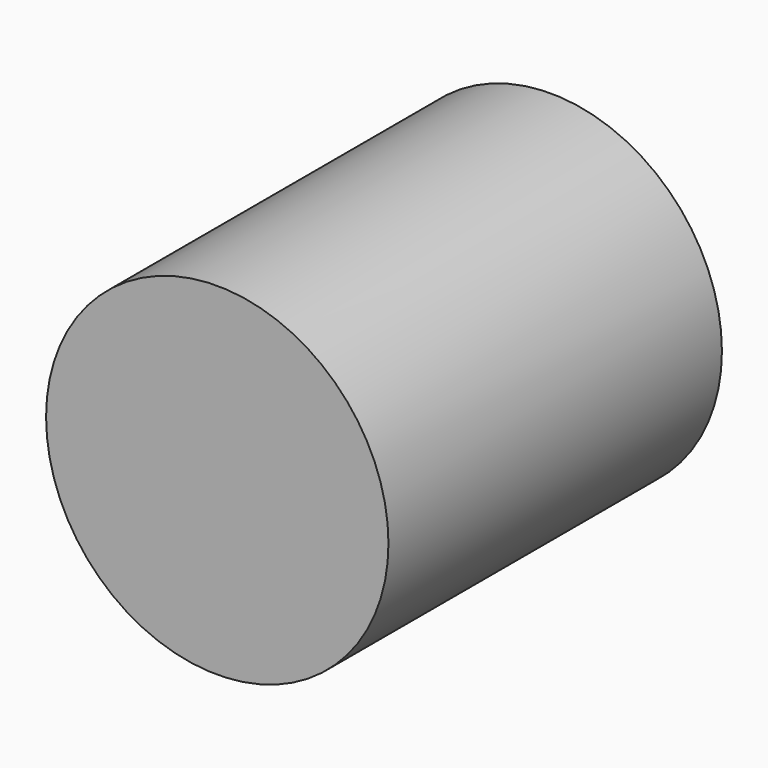
from build123d import *

# Parameters (mm, degrees)
F0_R     = 14.605
F0_R_2   = 1.016
F1_DEPTH = 35.56


# Not quite as in the source:
# - the program builds the solid bodies; features that only make, move or delete a surface that nothing else refers to are left out


with BuildPart() as f1:
    # F0 (on Front) → F1 (new body)
    with BuildSketch(Plane.XZ):
        with Locations((-19.2903056741, 14.9764399976)):
            Circle(F0_R)
        with Locations((-19.2903056741, 14.9764399976)):
            Circle(F0_R_2, mode=Mode.SUBTRACT)
        with Locations((-19.2903056741, 14.9764399976)):
            Circle(F0_R_2)
    extrude(amount=F1_DEPTH)


solid = f1.part
